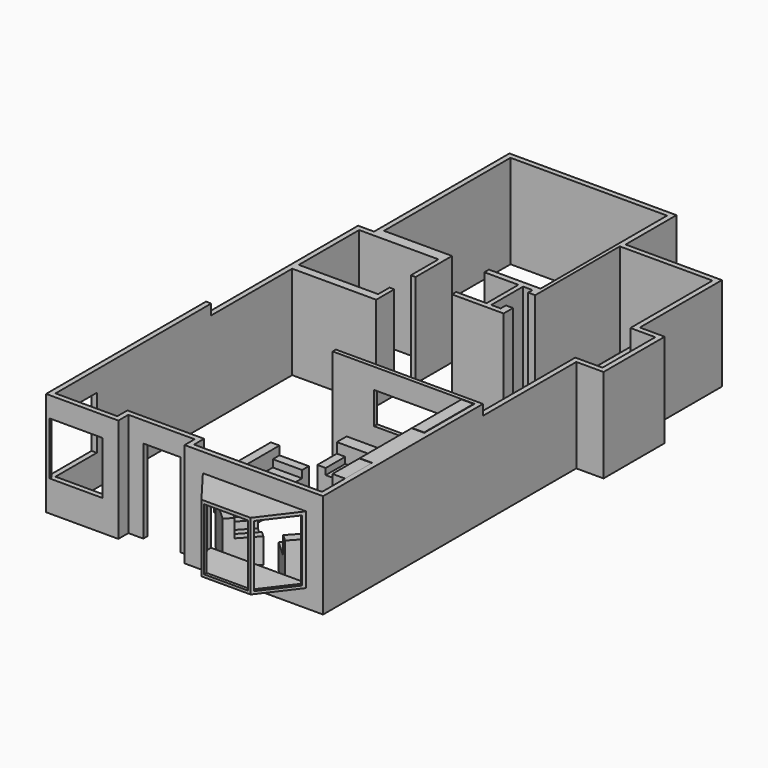
from build123d import *

# Parameters (mm, degrees)
F1_DEPTH  = 2527.3
F3_W      = 8943.5124397278
F3_H      = 9339.3726348877
F4_DEPTH  = 254
F5_W      = 1268.2032585144
F5_H      = 1822.1311569214
F6_DEPTH  = 1562.1
F7_W      = 304.8
F7_H      = 1574.8
F8_DEPTH  = 2527.3
F9_W      = 914.4
F9_H      = 457.2
F10_DEPTH = 152.4
F11_W     = 2311.4
F11_H     = 1587.5
F12_DEPTH = 127
F14_DEPTH = 1587.5
F16_DEPTH = 25.4
F18_DEPTH = 25.4
F19_W     = 1066.8
F19_H     = 1498.6
F20_DEPTH = 76.2
F21_W     = 937.2730590397
F21_H     = 1498.6
F22_DEPTH = 76.2
F23_W     = 937.2730590397
F23_H     = 1498.6
F24_DEPTH = 76.2
F25_W     = 901.7
F25_H     = 2032
F26_DEPTH = 127
F27_W     = 1282.7
F27_H     = 1282.7
F28_DEPTH = 127
F29_W     = 1282.7
F29_H     = 1282.7
F30_DEPTH = 127
F31_SIZE  = 43.18
F32_W     = 292.1
F32_H     = 1498.6
F33_DEPTH = 2527.3
F34_W     = 349.25
F34_H     = 609.6
F34_W_2   = 336.55
F34_H_2   = 596.9
F34_W_3   = 1397
F34_H_3   = 546.1
F34_H_4   = 355.6
F35_DEPTH = 292.1
F36_W     = 711.2
F36_H     = 355.6
F36_H_2   = 546.1
F37_DEPTH = 304.8
F38_W     = 635
F38_H     = 279.4
F38_W_2   = 355.6
F38_H_2   = 609.6
F38_W_3   = 342.9
F38_H_3   = 596.9
F39_DEPTH = 304.8
F40_W     = 2120.9
F40_H     = 774.7
F41_DEPTH = 98.425
F42_W     = 2438.4
F42_H     = 889
F43_DEPTH = 857.25
F45_DEPTH = 591.82
F46_W     = 920.75
F46_H     = 1720.85
F47_DEPTH = 793.75
F49_DEPTH = 711.2
F51_DEPTH = 1047.75
F53_DEPTH = 553.72
F55_ANGLE = 90


with BuildPart() as f1:
    # F0 (on Top) → F1 (new body)
    with BuildSketch(Plane.XY):
        Polygon((4311.65, 13436.6), (260.35, 13436.6), (260.35, 9332.109916687), (-127, 9332.109916687), (-127, -127), (1625.6, -127), (1625.6, 177.8), (3232.15, 177.8), (3232.15, -127), (6591.3, -127), (6591.3, 7550.15), (7251.7, 7550.15), (7251.7, 9404.35), (6648.45, 9404.35), (6648.45, 11893.55), (4311.65, 11893.55), align=None)
        Polygon((6464.3, 4622.8), (6464.3, 0), (3359.15, 0), (3359.15, 304.8), (1498.6, 304.8), (1498.6, 0), (0, 0), (0, 7175.5), (2038.35, 7175.5), (2038.35, 7721.6), (1924.05, 7721.6), (1924.05, 7376.309916687), (0, 7376.309916687), (0, 9205.109916687), (1924.05, 9205.109916687), (1924.05, 8369.3), (2038.35, 8369.3), (2038.35, 9474.2), (387.35, 9474.2), (387.35, 13309.6), (4184.65, 13309.6), (4184.65, 9474.2), (2933.7, 9474.2), (2933.7, 9334.5), (3759.2, 9334.5), (3759.2, 8369.3), (3022.6, 8369.3), (3022.6, 8242.3), (4273.55, 8242.3), (4273.55, 8528.05), (4102.1, 8528.05), (4102.1, 8369.3), (3873.5, 8369.3), (3873.5, 9334.5), (4102.1, 9334.5), (4102.1, 9201.15), (4273.55, 9201.15), (4273.55, 11766.55), (6521.45, 11766.55), (6521.45, 9417.05), (5562.6, 9417.05), (5562.6, 10801.35), (5435.6, 10801.35), (5435.6, 9277.35), (7124.7, 9277.35), (7124.7, 7677.15), (6464.3, 7677.15), (6464.3, 4721.225), (3581.4, 4721.225), (3581.4, 5076.825), (3143.25, 5076.825), (3143.25, 5051.425), (3022.6, 5051.425), (3022.6, 4622.8), align=None, mode=Mode.SUBTRACT)
    extrude(amount=F1_DEPTH)

    # F3 (on offset) → F4 (cut)
    with BuildSketch(Plane.XY.offset(2527.3)):
        with Locations((3140.6382170709, 9390.9113174438)):
            Rectangle(F3_W, F3_H)
    extrude(amount=-F4_DEPTH, mode=Mode.SUBTRACT)

    # F5 (on offset) → F6 (cut)
    with BuildSketch(Plane.XY.offset(2527.3)):
        with Locations((5887.3483707428, 10057.6597845367)):
            Rectangle(F5_W, F5_H)
    extrude(amount=-F6_DEPTH, mode=Mode.SUBTRACT)

    # F7 (on Top) → F8 (join)
    with BuildSketch(Plane.XY):
        with Locations((6311.9, 2311.4)):
            Rectangle(F7_W, F7_H)
    extrude(amount=F8_DEPTH)

    # F9 (on face) → F10 (cut)
    with BuildSketch(Plane(origin=(6159.5, 0, 0), x_dir=(0, -1, 0), z_dir=(-1, 0, 0))):
        with Locations((-2311.4, 609.6)):
            Rectangle(F9_W, F9_H)
    extrude(amount=-F10_DEPTH, mode=Mode.SUBTRACT)

    # F11 (on face) → F12 (cut, through all)
    with BuildSketch(Plane.XZ.offset(127)):
        with Locations((4927.6, 1250.95)):
            Rectangle(F11_W, F11_H)
    extrude(amount=-F12_DEPTH, mode=Mode.SUBTRACT)

    # F13 (on face) → F14 (join, through all)
    with BuildSketch(Plane.XY.offset(457.2)):
        Polygon((6083.3, -127), (5486.4, -914.4), (4368.8, -914.4), (3771.9, -127), (3676.2800265446, -127), (4330.9445426736, -990.6), (5524.2554573264, -990.6), (6178.9199734555, -127), align=None)
    extrude(amount=F14_DEPTH)

    # F15 (on face) → F16 (join)
    with BuildSketch(Plane.XY.offset(2044.7)):
        Polygon((6178.9199734555, -127), (3676.2800265446, -127), (4330.9445426736, -990.6), (5524.2554573264, -990.6), align=None)
    extrude(amount=F16_DEPTH)

    # F17 (on face) → F18 (join)
    with BuildSketch(Plane(origin=(0, 0, 457.2), x_dir=(1, 0, 0), z_dir=(0, 0, -1))):
        Polygon((4330.9445426736, 990.6), (3676.2800265446, 127), (6178.9199734555, 127), (5524.2554573264, 990.6), align=None)
    extrude(amount=F18_DEPTH)

    # F19 (on face) → F20 (cut, through all)
    with BuildSketch(Plane(origin=(0, -914.4, 0), x_dir=(-1, 0, 0), z_dir=(0, 1, 0))):
        with Locations((-4927.6, 1244.6)):
            Rectangle(F19_W, F19_H)
    extrude(amount=-F20_DEPTH, mode=Mode.SUBTRACT)

    # F21 (on face) → F22 (cut, through all)
    with BuildSketch(Plane(origin=(2334.2318850157, 1769.4983644474, 0), x_dir=(-0.6041051262, 0.7969046345, 0), z_dir=(0.7969046345, 0.6041051262, 0))):
        with Locations((-2873.8675435194, 1244.6)):
            Rectangle(F21_W, F21_H)
    extrude(amount=-F22_DEPTH, mode=Mode.SUBTRACT)

    # F23 (on face) → F24 (cut, through all)
    with BuildSketch(Plane(origin=(3924.3818271931, -2974.9346109367, 0), x_dir=(-0.6041051262, -0.7969046345, 0), z_dir=(-0.7969046345, 0.6041051262, 0))):
        with Locations((-3079.7092959478, 1244.6)):
            Rectangle(F23_W, F23_H)
    extrude(amount=-F24_DEPTH, mode=Mode.SUBTRACT)

    # F25 (on face) → F26 (cut, through all)
    with BuildSketch(Plane(origin=(0, 304.8, 0), x_dir=(-1, 0, 0), z_dir=(0, 1, 0))):
        with Locations((-2438.4, 1016)):
            Rectangle(F25_W, F25_H)
    extrude(amount=-F26_DEPTH, mode=Mode.SUBTRACT)

    # F27 (on face) → F28 (cut, through all)
    with BuildSketch(Plane(origin=(0, 0, 0), x_dir=(-1, 0, 0), z_dir=(0, 1, 0))):
        with Locations((-603.25, 1390.65)):
            Rectangle(F27_W, F27_H)
    extrude(amount=-F28_DEPTH, mode=Mode.SUBTRACT)

    # F29 (on face) → F30 (cut, through all)
    with BuildSketch(Plane.YZ):
        with Locations((609.6, 1390.65)):
            Rectangle(F29_W, F29_H)
    extrude(amount=-F30_DEPTH, mode=Mode.SUBTRACT)

    # F31
    f31_edges = [f1.edges().sort_by_distance(p)[0] for p in [
        (-38.1, -31.75, 1390.65),
    ]]
    chamfer(f31_edges, length=F31_SIZE)

    # F40 (on face) → F41 (cut, through all)
    with BuildSketch(Plane(origin=(0, 4721.225, 0), x_dir=(-1, 0, 0), z_dir=(0, 1, 0))):
        with Locations((-5086.35, 1644.65)):
            Rectangle(F40_W, F40_H)
    extrude(amount=-F41_DEPTH, mode=Mode.SUBTRACT)


with BuildPart() as f33:
    # F32 (on Top) → F33 (new body, through all)
    with BuildSketch(Plane.XY):
        with Locations((6305.55, 3860.8)):
            Rectangle(F32_W, F32_H)
    extrude(amount=F33_DEPTH)

    # F34 (on face) → F35 (cut, through all)
    with BuildSketch(Plane(origin=(6159.5, 0, 0), x_dir=(0, -1, 0), z_dir=(-1, 0, 0))):
        with Locations((-4384.675, 355.6)):
            Rectangle(F34_W, F34_H)
        with Locations((-4384.675, 355.6)):
            Rectangle(F34_W_2, F34_H_2, mode=Mode.SUBTRACT)
        with Locations((-4035.425, 355.6)):
            Rectangle(F34_W, F34_H)
        with Locations((-4035.425, 355.6)):
            Rectangle(F34_W_2, F34_H_2, mode=Mode.SUBTRACT)
        with Locations((-3686.175, 355.6)):
            Rectangle(F34_W, F34_H)
        with Locations((-3686.175, 355.6)):
            Rectangle(F34_W_2, F34_H_2, mode=Mode.SUBTRACT)
        with Locations((-3336.925, 355.6)):
            Rectangle(F34_W, F34_H)
        with Locations((-3336.925, 355.6)):
            Rectangle(F34_W_2, F34_H_2, mode=Mode.SUBTRACT)
        with Locations((-3860.8, 2203.45)):
            Rectangle(F34_W_3, F34_H_3)
        with Locations((-3860.8, 1701.8)):
            Rectangle(F34_W_3, F34_H_4)
        with Locations((-3860.8, 1295.4)):
            Rectangle(F34_W_3, F34_H_4)
        with Locations((-3860.8, 889)):
            Rectangle(F34_W_3, F34_H_4)
    extrude(amount=-F35_DEPTH, mode=Mode.SUBTRACT)


with BuildPart() as f37:
    # F36 (on face) → F37 (new body, through all)
    with BuildSketch(Plane(origin=(6464.3, 0, 0), x_dir=(0, -1, 0), z_dir=(-1, 0, 0))):
        Polygon((-698.5, 2527.3), (-1511.3, 2527.3), (-1511.3, 0), (-12.7, 0), (-12.7, 711.2), (-698.5, 711.2), align=None)
        with Locations((-1104.9, 889)):
            Rectangle(F36_W, F36_H, mode=Mode.SUBTRACT)
        with Locations((-1104.9, 1295.4)):
            Rectangle(F36_W, F36_H, mode=Mode.SUBTRACT)
        with Locations((-1104.9, 1701.8)):
            Rectangle(F36_W, F36_H, mode=Mode.SUBTRACT)
        with Locations((-1104.9, 2203.45)):
            Rectangle(F36_W, F36_H_2, mode=Mode.SUBTRACT)
    extrude(amount=F37_DEPTH)

    # F38 (on face) → F39 (cut, through all)
    with BuildSketch(Plane(origin=(6159.5, 0, 0), x_dir=(0, -1, 0), z_dir=(-1, 0, 0))):
        with Locations((-381, 520.7)):
            Rectangle(F38_W, F38_H)
        with Locations((-381, 190.5)):
            Rectangle(F38_W, F38_H)
        with Locations((-1282.7, 355.6)):
            Rectangle(F38_W_2, F38_H_2)
        with Locations((-1282.7, 355.6)):
            Rectangle(F38_W_3, F38_H_3, mode=Mode.SUBTRACT)
        with Locations((-927.1, 355.6)):
            Rectangle(F38_W_2, F38_H_2)
        with Locations((-927.1, 355.6)):
            Rectangle(F38_W_3, F38_H_3, mode=Mode.SUBTRACT)
    extrude(amount=-F39_DEPTH, mode=Mode.SUBTRACT)


with BuildPart() as f43:
    # F42 (on Top) → F43 (new body)
    with BuildSketch(Plane.XY):
        with Locations((4622.8, 4127.5)):
            Rectangle(F42_W, F42_H)
    extrude(amount=F43_DEPTH)

    # F44 (on face) → F45 (cut)
    with BuildSketch(Plane.XZ.offset(-3683)):
        Polygon((3403.6, 857.25), (3403.6, 609.6), (3606.8, 609.6), (3606.8, 457.2), (5638.8, 457.2), (5638.8, 609.6), (5842, 609.6), (5842, 857.25), align=None)
    extrude(amount=-F45_DEPTH, mode=Mode.SUBTRACT)


with BuildPart() as f47:
    # F46 (on Top) → F47 (new body)
    with BuildSketch(Plane.XY):
        with Locations((2818.3227291107, 2720.6609203339)):
            Rectangle(F46_W, F46_H)
    extrude(amount=F47_DEPTH)

    # F48 (on face) → F49 (cut)
    with BuildSketch(Plane.YZ.offset(3278.6977291107)):
        Polygon((1860.2359203339, 793.75), (1860.2359203339, 584.2), (2063.4359203339, 584.2), (2063.4359203339, 406.4), (3377.8859203339, 406.4), (3377.8859203339, 584.2), (3581.0859203339, 584.2), (3581.0859203339, 793.75), align=None)
    extrude(amount=-F49_DEPTH, mode=Mode.SUBTRACT)


with BuildPart() as f51:
    # F50 (on Top) → F51 (new body)
    with BuildSketch(Plane.XY):
        Polygon((4543.5538291931, 747.2482919693), (3909.8777690643, 1324.5975911978), (3383.848407545, 747.2482919693), (4017.5244676738, 169.8989927408), align=None)
    extrude(amount=F51_DEPTH)


with BuildPart() as f51b:
    # F50 (on Top) → F51, piece 2 (new body)
    with BuildSketch(Plane.XY):
        Polygon((5391.092300415, 221.21893045), (5968.4415996435, 854.8949905789), (5391.092300415, 1380.9243520981), (4813.7430011866, 747.2482919693), align=None)
    extrude(amount=F51_DEPTH)

    # F52 (on face) → F53 (cut)
    with BuildSketch(Plane(origin=(2258.2721205395, -2057.536820936, 0), x_dir=(-0.6734899962, -0.7391963373, 0), z_dir=(-0.7391963373, 0.6734899962, 0))):
        Polygon((-4651.620955957, 1047.75), (-4651.620955957, 609.6), (-4473.820955957, 609.6), (-4473.820955957, 431.8), (-3972.170955957, 431.8), (-3972.170955957, 609.6), (-3794.370955957, 609.6), (-3794.370955957, 1047.75), align=None)
    extrude(amount=-F53_DEPTH, mode=Mode.SUBTRACT)


with BuildPart() as f55_1:
    # F55: copy of F51b
    add(f51b.part.rotate(Axis((3359.15, 304.8, 1263.65), (0, 0, -1)), F55_ANGLE))


with BuildPart() as f55_1_1:
    # F56: moved
    add(f55_1.part.moved(Location((0, 2486.66, 0))))


solid = Compound([f1.part, f33.part, f37.part, f43.part, f47.part, f51b.part, f55_1_1.part])
